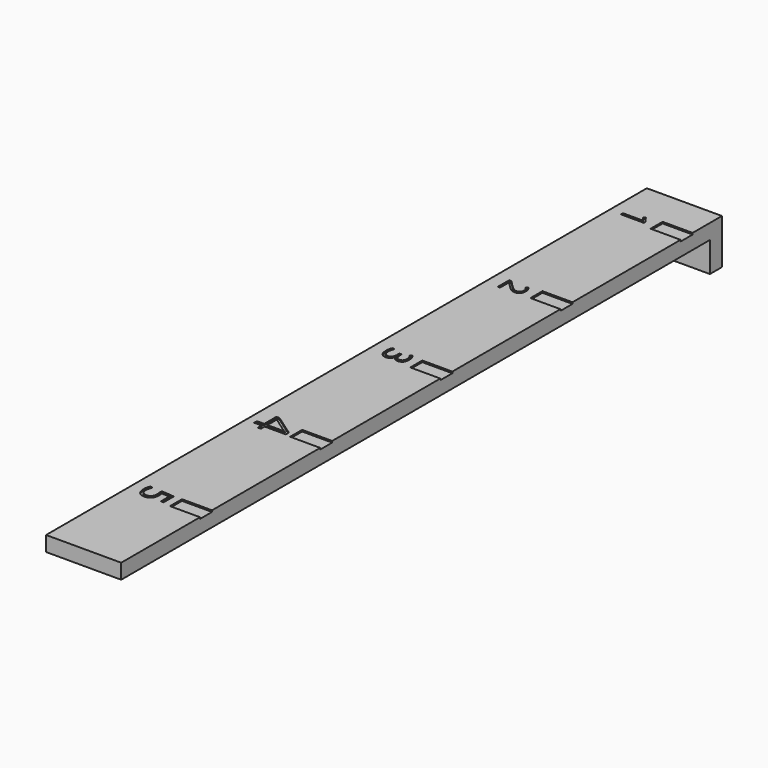
from build123d import *

# Parameters (mm, degrees)
F0_W           = 5
F0_H           = 50
F1_DEPTH       = 1
F2_W           = 5
F2_H           = 1
F3_DEPTH       = 2
F4_W           = 2
F4_H           = 1
F5_DEPTH       = 0.1
F6_TEXT_SIZE   = 2.146165611
F6_TEXT_SIZE_2 = 2.0234250567
F6_TEXT_SIZE_3 = 2.1741285713
F6_TEXT_SIZE_4 = 2.9303456864
F6_TEXT_SIZE_5 = 2.4104453284
F7_DEPTH       = 0.1


# Not quite as in the source:
# - Text() gives the source's letters only with a copy of the font that has no kerning and outlines rounded to 1/6400 em; it was checked with that copy


with BuildPart() as f1:
    # F0 (on Top) → F1 (new body)
    with BuildSketch(Plane.XY):
        with Locations((-31.1472881585, 13.4895758893)):
            Rectangle(F0_W, F0_H)
    extrude(amount=F1_DEPTH)

    # F2 (on face) → F3 (join)
    with BuildSketch(Plane(origin=(0, 0, 0), x_dir=(1, 0, 0), z_dir=(0, 0, -1))):
        with Locations((-31.1472881585, -37.9895758893)):
            Rectangle(F2_W, F2_H)
    extrude(amount=F3_DEPTH)

    # F4 (on face) → F5 (cut)
    with BuildSketch(Plane.XY.offset(1)):
        with Locations((-29.6472881585, 35.5509231687)):
            Rectangle(F4_W, F4_H)
        with Locations((-29.6472881585, 25.5509231687)):
            Rectangle(F4_W, F4_H)
        with Locations((-29.6472881585, 15.5509231687)):
            Rectangle(F4_W, F4_H)
        with Locations((-29.6472881585, 5.5509231687)):
            Rectangle(F4_W, F4_H)
        with Locations((-29.6472881585, -4.4490768313)):
            Rectangle(F4_W, F4_H)
    extrude(amount=-F5_DEPTH, mode=Mode.SUBTRACT)

    # F6 (on face) → F7 (cut)
    with BuildSketch(Plane.XY.offset(1)):
        with Locations(Location((-32.8630944156, 36.0976169444), (0, 0, -90))):
            Text('1', F6_TEXT_SIZE, font='Open Sans', text_align=(TextAlign.LEFT, TextAlign.BOTTOM))
        with Locations(Location((-32.7650728096, 26.0308915357), (0, 0, -90))):
            Text('2', F6_TEXT_SIZE_2, font='Open Sans', text_align=(TextAlign.LEFT, TextAlign.BOTTOM))
        with Locations(Location((-32.7924650592, 16.2636607456), (0, 0, -90))):
            Text('3', F6_TEXT_SIZE_3, font='Open Sans', text_align=(TextAlign.LEFT, TextAlign.BOTTOM))
        with Locations(Location((-33.090511655, 6.4243885301), (0, 0, -90))):
            Text('4', F6_TEXT_SIZE_4, font='Open Sans', text_align=(TextAlign.LEFT, TextAlign.BOTTOM))
        with Locations(Location((-32.8926861052, -3.710527229), (0, 0, -90))):
            Text('5', F6_TEXT_SIZE_5, font='Open Sans', text_align=(TextAlign.LEFT, TextAlign.BOTTOM))
    extrude(amount=-F7_DEPTH, mode=Mode.SUBTRACT)


solid = f1.part
